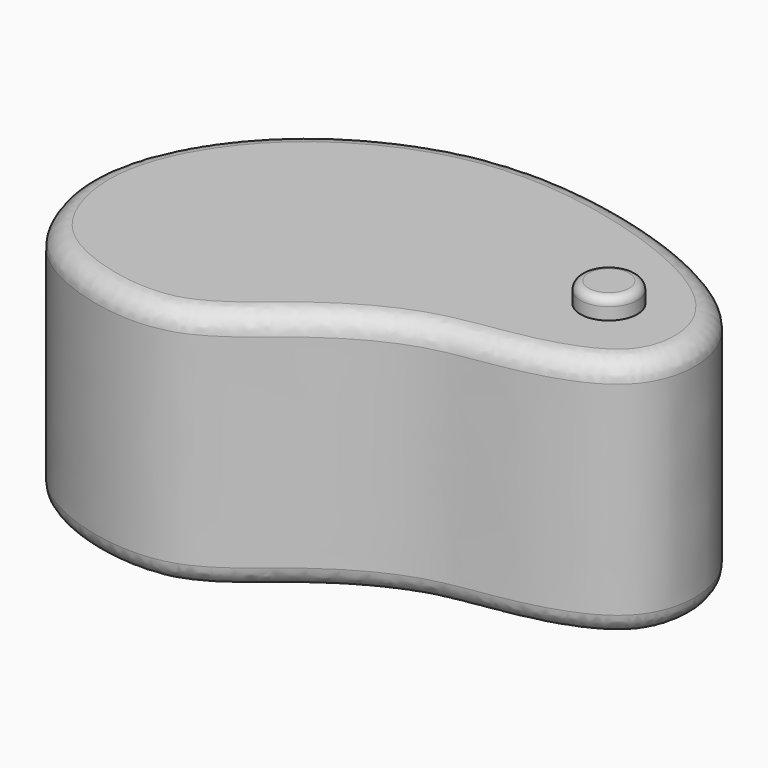
from build123d import *

# Parameters (mm, degrees)
F1_DEPTH = 60
F2_R     = 5
F3_R     = 7
F4_DEPTH = 5
F5_R     = 2


with BuildPart() as f1:
    # F0 (on Top) → F1 (new body)
    with BuildSketch(Plane.XY):
        with BuildLine():
            add(Edge.make_bspline(
                [(46.6075725853, 0), (37.6135667066, -2.2337441277), (17.2080035039, 2.2439024187), (3.8657979354, 14.5964755975), (-1.5166241531, 33.023539869), (2.2732014922, 51.8180100869), (15.4936104431, 71.1166405023), (37.7712487652, 86.1339923735), (72.0238414784, 94.05332559), (123.3038555539, 78.4121603646), (137.4838253152, 57.0911804312), (133.3338393023, 35.7314392459), (108.3258257585, 27.9351395013), (88.6557729057, 26.6263742062), (67.5094921509, 14.5917224807), (55.1347572905, 2.1178047933), (46.6075725853, 0)],
                knots=[0, 0, 0, 0, 0.0772175705, 0.137765267, 0.1986611263, 0.2608564904, 0.3294823599, 0.4026900719, 0.4881255596, 0.59189909, 0.6610271706, 0.7216628246, 0.7920782139, 0.8569002959, 0.9267902984, 1, 1, 1, 1], degree=3))
        make_face()
    extrude(amount=F1_DEPTH)

    # F2
    f2_edges = [f1.edges().sort_by_distance(p)[0] for p in [
        (82.294885, 88.796047, 60),
        (82.294885, 88.796047, 0),
    ]]
    fillet(f2_edges, radius=F2_R)

    # F3 (on face) → F4 (join)
    with BuildSketch(Plane.XY.offset(60)):
        with Locations((112.1847704053, 54.2634055018)):
            Circle(F3_R)
    extrude(amount=F4_DEPTH)

    # F5
    f5_edges = [f1.edges().sort_by_distance(p)[0] for p in [
        (105.18477, 54.263406, 65),
    ]]
    fillet(f5_edges, radius=F5_R)


solid = f1.part
